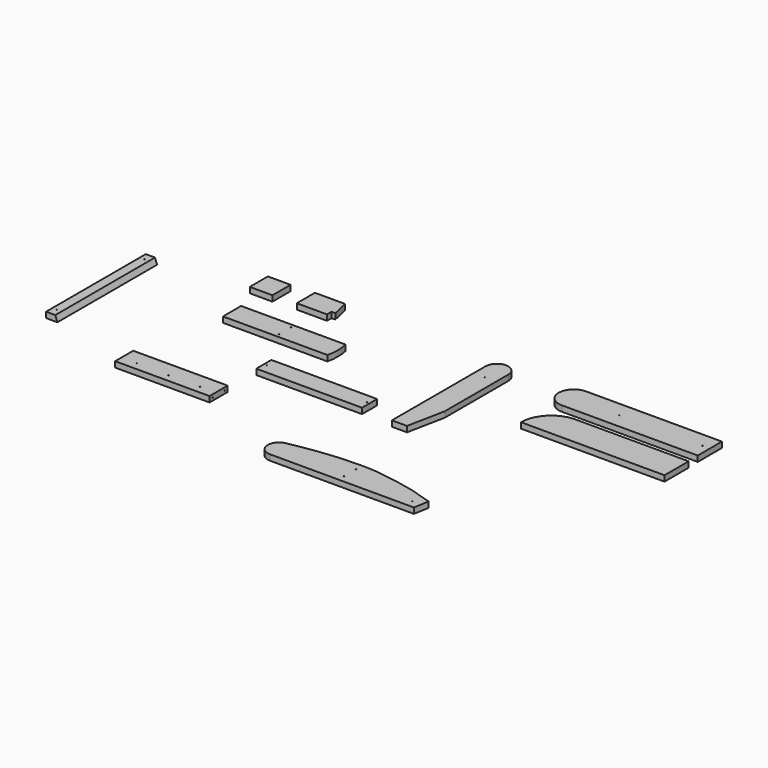
from build123d import *

# Parameters (mm, degrees)
F0_R      = 1.27
F1_DEPTH  = 19.05
F4_R      = 1.27
F5_DEPTH  = 19.05
F6_R      = 1.27
F7_DEPTH  = 19.05
F8_R      = 1.27
F9_DEPTH  = 19.05
F10_R     = 1.27
F11_DEPTH = 19.05
F13_DEPTH = 419.1
F14_R     = 1.27
F15_DEPTH = 19.05
F16_R     = 1.27
F17_DEPTH = 19.05
F18_W     = 76.2
F18_H     = 76.2
F19_DEPTH = 19.05
F21_DEPTH = 19.05
F26_DEPTH = 19.05
F27_R     = 1.27
F28_DEPTH = 19.05
F29_R     = 1.27
F30_DEPTH = 19.05
F31_R     = 1.27
F32_DEPTH = 19.05


# Not quite as in the source:
# - the program builds the solid bodies; features that only make, move or delete a surface that nothing else refers to are left out


with BuildPart() as f1:
    # F0 (on Top) → F1 (new body)
    with BuildSketch(Plane.XY):
        with BuildLine():
            Line((-60.932392, 59.310776), (-60.932392, -334.389224))
            Line((-60.932392, -334.389224), (-10.132392, -334.389224))
            Line((-10.132392, -334.389224), (15.267608, -207.389224))
            Line((15.267608, -207.389224), (15.267608, 59.310776))
            ThreePointArc((15.267608, 59.310776), (4.108376, 86.251544), (-22.832392, 97.410776))
            ThreePointArc((-22.832392, 97.410776), (-49.773161, 86.251544), (-60.932392, 59.310776))
        make_face()
        with Locations((-35.532392, -315.339224)):
            Circle(F0_R, mode=Mode.SUBTRACT)
        with BuildLine():
            ThreePointArc((-22.832392, 9.780776), (-21.934367, 9.408801), (-21.562392, 8.510776))
            ThreePointArc((-21.562392, 8.510776), (-23.730418, 7.61275), (-22.832392, 9.780776))
        make_face(mode=Mode.SUBTRACT)
    extrude(amount=F1_DEPTH)


with BuildPart() as f2_1:
    # F2: copy of F1
    add(f1.part.moved(Location((812.8, 0, 0))))


with BuildPart() as f5:
    # F4 (on Top) → F5 (new body)
    with BuildSketch(Plane.XY):
        with BuildLine():
            Line((210.500181, -131.009649), (693.100181, -131.009649))
            Line((693.100181, -131.009649), (693.100181, -80.209649))
            Line((693.100181, -80.209649), (693.100181, -29.409649))
            Line((693.100181, -29.409649), (312.100181, -29.409649))
            ThreePointArc((312.100181, -29.409649), (240.258132, -59.167601), (210.500181, -131.009649))
        make_face()
        with Locations((667.700181, -80.209649)):
            Circle(F4_R, mode=Mode.SUBTRACT)
    extrude(amount=F5_DEPTH)


with BuildPart() as f7:
    # F6 (on Top) → F7 (new body)
    with BuildSketch(Plane.XY):
        with BuildLine():
            Line((233.91931, 11.164315), (691.11931, 11.164315))
            Line((691.11931, 11.164315), (691.11931, 61.964315))
            Line((691.11931, 61.964315), (691.11931, 112.764315))
            Line((691.11931, 112.764315), (233.91931, 112.764315))
            ThreePointArc((233.91931, 112.764315), (269.840334, 97.88534), (284.71931, 61.964315))
            ThreePointArc((284.71931, 61.964315), (269.840334, 26.043291), (233.91931, 11.164315))
        make_face()
        with Locations((386.31931, 61.964315)):
            Circle(F6_R, mode=Mode.SUBTRACT)
        with Locations((665.71931, 61.964315)):
            Circle(F6_R, mode=Mode.SUBTRACT)
        with BuildLine():
            Line((233.91931, 112.764315), (233.91931, 11.164315))
            ThreePointArc((233.91931, 11.164315), (269.840334, 26.043291), (284.71931, 61.964315))
            ThreePointArc((284.71931, 61.964315), (269.840334, 97.88534), (233.91931, 112.764315))
        make_face()
        with BuildLine():
            ThreePointArc((233.91931, 112.764315), (183.11931, 61.964315), (233.91931, 11.164315))
            Line((233.91931, 11.164315), (233.91931, 112.764315))
        make_face()
    extrude(amount=F7_DEPTH)


with BuildPart() as f9:
    # F8 (on Top) → F9 (new body)
    with BuildSketch(Plane.XY):
        with BuildLine():
            ThreePointArc((-192.656518, -609.057055), (-228.063516, -648.512913), (-189.759585, -685.163002))
            Line((-189.759585, -685.163002), (39.529742, -685.163002))
            Line((39.529742, -685.163002), (39.529742, -662.13299))
            ThreePointArc((39.529742, -662.13299), (38.259742, -660.86299), (39.529742, -659.59299))
            Line((39.529742, -659.59299), (39.529742, -611.33299))
            ThreePointArc((39.529742, -611.33299), (38.259742, -610.06299), (39.529742, -608.79299))
            Line((39.529742, -608.79299), (39.529742, -584.66299))
            add(Edge.make_bspline(
                [(39.529742, -584.66299), (8.240435, -584.48981), (-69.693829, -586.989314), (-164.102703, -603.394447), (-192.656518, -609.057055)],
                knots=[0.566257, 0.566257, 0.566257, 0.566257, 0.77812, 1, 1, 1, 1], degree=3))
        make_face()
        with BuildLine():
            Line((39.529742, -662.13299), (39.529742, -685.163002))
            Line((39.529742, -685.163002), (293.529742, -685.163002))
            Line((293.529742, -685.163002), (302.649135, -634.363002))
            add(Edge.make_bspline(
                [(302.649135, -634.363002), (272.109092, -624.904008), (239.994661, -612.093395), (113.364797, -587.287349), (65.492526, -584.806689), (39.529742, -584.66299)],
                knots=[0.000416, 0.000416, 0.000416, 0.000416, 0.171079, 0.390461, 0.566257, 0.566257, 0.566257, 0.566257], degree=3))
            Line((39.529742, -584.66299), (39.529742, -608.79299))
            ThreePointArc((39.529742, -608.79299), (40.427768, -609.164964), (40.799742, -610.06299))
            ThreePointArc((40.799742, -610.06299), (40.427768, -610.961016), (39.529742, -611.33299))
            Line((39.529742, -611.33299), (39.529742, -659.59299))
            ThreePointArc((39.529742, -659.59299), (40.427768, -659.964964), (40.799742, -660.86299))
            ThreePointArc((40.799742, -660.86299), (40.427768, -661.761016), (39.529742, -662.13299))
        make_face()
        with Locations((267.440415, -659.763002)):
            Circle(F8_R, mode=Mode.SUBTRACT)
    extrude(amount=F9_DEPTH)


with BuildPart() as f11:
    # F10 (on Top) → F11 (new body)
    with BuildSketch(Plane.XY):
        Polygon((-838.564605, -500.333173), (-838.564605, -525.733173), (-679.814605, -525.733173), (-521.064605, -525.733173), (-521.064605, -449.533173), (-838.564605, -449.533173), align=None)
        with Locations((-786.546743, -500.333173)):
            Circle(F10_R, mode=Mode.SUBTRACT)
        with BuildLine():
            ThreePointArc((-678.596743, -500.333173), (-678.950469, -501.212571), (-679.814605, -501.602102))
            ThreePointArc((-679.814605, -501.602102), (-680.746142, -501.249447), (-681.136743, -500.333173))
            ThreePointArc((-681.136743, -500.333173), (-680.746142, -499.416899), (-679.814605, -499.064244))
            ThreePointArc((-679.814605, -499.064244), (-678.950469, -499.453774), (-678.596743, -500.333173))
        make_face(mode=Mode.SUBTRACT)
        with Locations((-573.186743, -500.333173)):
            Circle(F10_R, mode=Mode.SUBTRACT)
    extrude(amount=F11_DEPTH)

    # F27 (on face) → F28 (cut)
    with BuildSketch(Plane(origin=(-838.564605, 0, 0), x_dir=(0, -1, 0), z_dir=(-1, 0, 0))):
        with Locations((462.233173, 9.525)):
            Circle(F27_R)
        with Locations((513.033173, 9.525)):
            Circle(F27_R)
    extrude(amount=-F28_DEPTH, mode=Mode.SUBTRACT)

    # F29 (on face) → F30 (cut)
    with BuildSketch(Plane.YZ.offset(-521.064605)):
        with Locations((-462.233173, 9.525)):
            Circle(F29_R)
        with BuildLine():
            ThreePointArc((-514.303173, 9.525), (-513.033173, 8.255), (-511.763173, 9.525))
            ThreePointArc((-511.763173, 9.525), (-513.033173, 10.795), (-514.303173, 9.525))
        make_face()
    extrude(amount=-F30_DEPTH, mode=Mode.SUBTRACT)


with BuildPart() as f13:
    # F12 (on Front) → F13 (new body)
    with BuildSketch(Plane.XZ):
        Polygon((-1156.008205, 19.05), (-1156.008205, 0), (-1117.908205, 0), (-1125.008583, 19.05), align=None)
    extrude(amount=F13_DEPTH)

    # F25 (on face) → F26 (cut)
    with BuildSketch(Plane.XY.offset(19.05)):
        with BuildLine():
            ThreePointArc((-1140.508394, -394.97), (-1139.610369, -394.598026), (-1139.238394, -393.7))
            ThreePointArc((-1139.238394, -393.7), (-1141.40642, -392.801974), (-1140.508394, -394.97))
        make_face()
        with BuildLine():
            ThreePointArc((-1140.508394, -24.13), (-1141.40642, -26.298026), (-1139.238394, -25.4))
            ThreePointArc((-1139.238394, -25.4), (-1139.610369, -24.501974), (-1140.508394, -24.13))
        make_face()
    extrude(amount=-F26_DEPTH, mode=Mode.SUBTRACT)


with BuildPart() as f15:
    # F14 (on Top) → F15 (new body)
    with BuildSketch(Plane.XY):
        Polygon((-522.584672, -263.863193), (-522.584672, -327.363193), (-166.984672, -327.363193), (-166.984672, -295.613193), (-166.984672, -263.863193), align=None)
        with Locations((-512.805672, -295.613193)):
            Circle(F14_R, mode=Mode.SUBTRACT)
        with Locations((-176.255672, -295.613193)):
            Circle(F14_R, mode=Mode.SUBTRACT)
    extrude(amount=F15_DEPTH)

    # F31 (on face) → F32 (cut)
    with BuildSketch(Plane(origin=(-522.584672, 0, 0), x_dir=(0, -1, 0), z_dir=(-1, 0, 0))):
        with Locations((295.613193, 9.525)):
            Circle(F31_R)
    extrude(amount=-F32_DEPTH, mode=Mode.SUBTRACT)


with BuildPart() as f17:
    # F16 (on Top) → F17 (new body)
    with BuildSketch(Plane.XY):
        with BuildLine():
            Line((-424.947367, -73.803925), (-776.417255, -73.803925))
            Line((-776.417255, -73.803925), (-776.417255, -150.003925))
            Line((-776.417255, -150.003925), (-598.617255, -150.003925))
            Line((-598.617255, -150.003925), (-424.947367, -150.003925))
            ThreePointArc((-424.947367, -150.003925), (-420.817255, -111.903925), (-424.947367, -73.803925))
        make_face()
        with BuildLine():
            ThreePointArc((-597.347255, -137.303925), (-597.71923, -138.201951), (-598.617255, -138.573925))
            ThreePointArc((-598.617255, -138.573925), (-599.515281, -136.405899), (-597.347255, -137.303925))
        make_face(mode=Mode.SUBTRACT)
        with Locations((-598.617255, -86.503925)):
            Circle(F16_R, mode=Mode.SUBTRACT)
    extrude(amount=F17_DEPTH)


with BuildPart() as f19:
    # F18 (on Top) → F19 (new body)
    with BuildSketch(Plane.XY):
        with Locations((-788.341646, 63.181495)):
            Rectangle(F18_W, F18_H)
    extrude(amount=F19_DEPTH)


with BuildPart() as f21:
    # F20 (on Top) → F21 (new body)
    with BuildSketch(Plane.XY):
        Polygon((-570.377707, 105.829176), (-671.977707, 105.829176), (-671.977707, 29.629176), (-570.377707, 29.629176), (-570.377707, 48.679176), (-557.677707, 48.679176), align=None)
    extrude(amount=F21_DEPTH)


solid = Compound([f1.part, f5.part, f7.part, f9.part, f11.part, f13.part, f15.part, f17.part, f19.part, f21.part])
